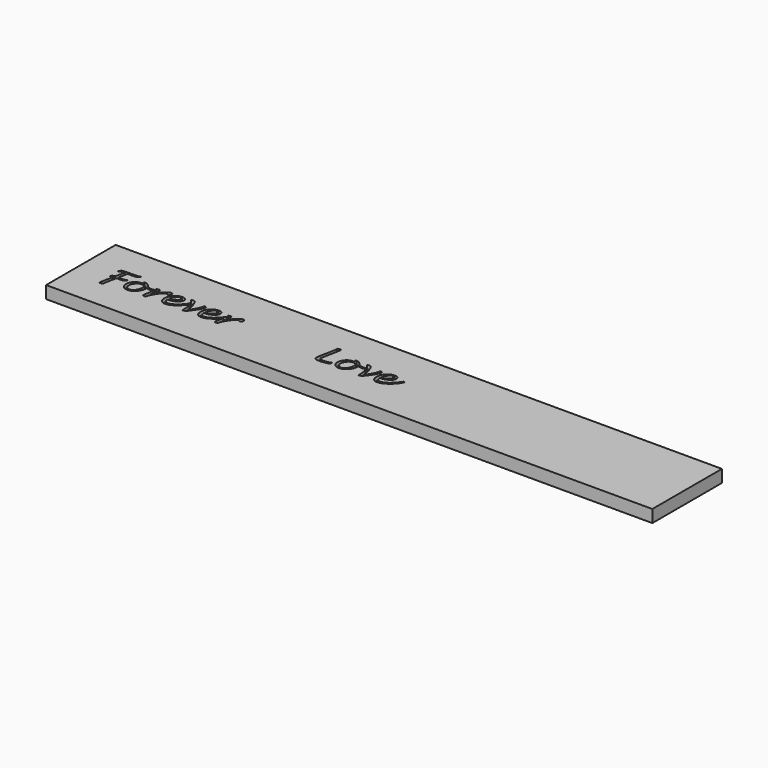
from build123d import *

# Parameters (mm, degrees)
F0_W     = 774.7
F0_H     = 111.125
F1_DEPTH = 15.875
F3_DEPTH = 4.7625


# Not quite as in the source:
# - ends of sketch curves that miss each other by under 0.0002 mm in the source are joined


with BuildPart() as f1:
    # F0 (on Top) → F1 (new body)
    with BuildSketch(Plane.XY):
        with Locations((387.35, 55.5625)):
            Rectangle(F0_W, F0_H)
    extrude(amount=F1_DEPTH)

    # F2 (on face) → F3 (cut)
    with BuildSketch(Plane.XY.offset(15.875)):
        with BuildLine():
            add(Edge.make_bspline(
                [(42.8841666709, 41.7124110682), (42.6348402709, 40.4654742682), (42.5101770709, 39.6582368682), (42.5101770709, 39.2906988682)],
                knots=[0, 0, 0, 0, 1, 1, 1, 1], degree=3))
            Line((42.8841666709, 41.7124110682), (45.6012046709, 55.3173368682))
            Line((45.6012046709, 55.3173368682), (49.8541806709, 55.3177940682))
            add(Edge.make_bspline(
                [(54.6779454709, 55.9281052682), (53.8641548709, 55.5212226682), (52.2562078709, 55.3177940682), (49.8541806709, 55.3177940682)],
                knots=[0, 0, 0, 0, 1, 1, 1, 1], degree=3))
            add(Edge.make_bspline(
                [(56.8633868709, 58.7633040682), (56.2333398709, 57.2800964682), (55.5048678709, 56.3350386682), (54.6779454709, 55.9281052682)],
                knots=[0, 0, 0, 0, 1, 1, 1, 1], degree=3))
            add(Edge.make_bspline(
                [(50.3266968709, 57.7591658682), (52.9649948709, 57.7591658682), (55.1438830709, 58.0938616682), (56.8633868709, 58.7633040682)],
                knots=[0, 0, 0, 0, 1, 1, 1, 1], degree=3))
            Line((50.3266968709, 57.7591658682), (46.0739240709, 57.7591658682))
            Line((46.0739240709, 57.7591658682), (48.4169216709, 69.5330310682))
            Line((48.4169216709, 69.5330310682), (54.4416492709, 69.5330310682))
            Line((54.4416492709, 69.5330310682), (56.1742594709, 69.5128634682))
            add(Edge.make_bspline(
                [(60.2498164709, 70.2216758682), (59.3704176709, 69.7491342682), (58.0118986709, 69.5128634682), (56.1742594709, 69.5128634682)],
                knots=[0, 0, 0, 0, 1, 1, 1, 1], degree=3))
            add(Edge.make_bspline(
                [(62.8093744709, 73.0962192682), (61.9955838709, 71.6655134682), (61.1423978709, 70.7073492682), (60.2498164709, 70.2216758682)],
                knots=[0, 0, 0, 0, 1, 1, 1, 1], degree=3))
            add(Edge.make_bspline(
                [(53.1815806709, 72.0724468682), (57.0405772709, 72.0724468682), (60.2498418709, 72.4136958682), (62.8093744709, 73.0962192682)],
                knots=[0, 0, 0, 0, 1, 1, 1, 1], degree=3))
            Line((53.1815806709, 72.0724468682), (48.0034604709, 72.0724468682))
            add(Edge.make_bspline(
                [(39.6948156709, 71.3439494682), (40.5873462709, 71.8296228682), (43.3569114709, 72.0724468682), (48.0034604709, 72.0724468682)],
                knots=[0, 0, 0, 0, 1, 1, 1, 1], degree=3))
            add(Edge.make_bspline(
                [(37.0368580709, 67.1896270682), (37.5487442709, 69.2634862682), (38.4347470709, 70.6482688682), (39.6948156709, 71.3439494682)],
                knots=[0, 0, 0, 0, 1, 1, 1, 1], degree=3))
            add(Edge.make_bspline(
                [(43.8687976709, 69.5325738682), (41.0073860709, 69.5325738682), (38.7300728709, 68.7516000682), (37.0368580709, 67.1896270682)],
                knots=[0, 0, 0, 0, 1, 1, 1, 1], degree=3))
            Line((43.8687976709, 69.5325738682), (44.3017660709, 69.5325738682))
            Line((44.3017660709, 69.5325738682), (41.9391088709, 57.7587086682))
            Line((41.9391088709, 57.7587086682), (41.4075122709, 57.7587086682))
            add(Edge.make_bspline(
                [(39.0448804709, 57.1483720682), (39.5436602709, 57.5552546682), (40.3312126709, 57.7587086682), (41.4075122709, 57.7587086682)],
                knots=[0, 0, 0, 0, 1, 1, 1, 1], degree=3))
            add(Edge.make_bspline(
                [(37.3516656709, 54.4707040682), (37.9948190709, 55.8620398682), (38.5592070709, 56.7545958682), (39.0448804709, 57.1483720682)],
                knots=[0, 0, 0, 0, 1, 1, 1, 1], degree=3))
            add(Edge.make_bspline(
                [(41.1712668709, 55.3173368682), (39.9899636709, 55.3173368682), (38.7167632709, 55.0351174682), (37.3516656709, 54.4707040682)],
                knots=[0, 0, 0, 0, 1, 1, 1, 1], degree=3))
            Line((41.1712668709, 55.3173368682), (41.4666434709, 55.3173368682))
            Line((41.4666434709, 55.3173368682), (38.4936496709, 40.3735516682))
            add(Edge.make_bspline(
                [(38.1000004709, 37.9321798682), (38.1000004709, 38.2208254682), (38.2312168709, 39.0346160682), (38.4936496709, 40.3735516682)],
                knots=[0, 0, 0, 0, 1, 1, 1, 1], degree=3))
            add(Edge.make_bspline(
                [(39.1238490709, 37.1052828682), (38.4413002709, 37.1052828682), (38.1000004709, 37.3808982682), (38.1000004709, 37.9321798682)],
                knots=[0, 0, 0, 0, 1, 1, 1, 1], degree=3))
            add(Edge.make_bspline(
                [(42.7662344709, 38.1093956682), (41.4405322709, 37.4399786682), (40.2264122709, 37.1052828682), (39.1238490709, 37.1052828682)],
                knots=[0, 0, 0, 0, 1, 1, 1, 1], degree=3))
            add(Edge.make_bspline(
                [(42.5101770709, 39.2906988682), (42.5101770709, 38.9231862682), (42.5955210709, 38.5294354682), (42.7662344709, 38.1093956682)],
                knots=[0, 0, 0, 0, 1, 1, 1, 1], degree=3))
        make_face()
        with BuildLine():
            add(Edge.make_bspline(
                [(82.6554564739, 57.4433294306), (82.6947450052, 57.1286193013), (82.7143892709, 56.8465227238), (82.7143892709, 56.5970650682)],
                knots=[0.0003900722, 0.0003900722, 0.0003900722, 0.0003900722, 1, 1, 1, 1], degree=3))
            add(Edge.make_bspline(
                [(87.6166400709, 56.5377814682), (86.1597881245, 56.5377814682), (84.5060602589, 56.8396477192), (82.6554564739, 57.4433294306)],
                knots=[0, 0, 0, 0, 0.9999368173, 0.9999368173, 0.9999368173, 0.9999368173], degree=3))
            add(Edge.make_bspline(
                [(91.5525691041, 57.3439651685), (90.2599710329, 56.8065131621), (88.9479984823, 56.5377814682), (87.6166400709, 56.5377814682)],
                knots=[0.3926410414, 0.3926410414, 0.3926410414, 0.3926410414, 1, 1, 1, 1], degree=3))
            add(Edge.make_bspline(
                [(91.5525691041, 57.3439651685), (91.6859533121, 58.2821458932), (91.7633692368, 59.0804045786), (91.7848148506, 59.7387412247)],
                knots=[0.4869393533, 0.4869393533, 0.4869393533, 0.4869393533, 0.9175112155, 0.9175112155, 0.9175112155, 0.9175112155], degree=3))
            add(Edge.make_bspline(
                [(88.0695220709, 58.8413582682), (89.2360031141, 58.8413582682), (90.4744377518, 59.1404859201), (91.7848148529, 59.7387412239)],
                knots=[0, 0, 0, 0, 0.7595714679, 0.7595714679, 0.7595714679, 0.7595714679], degree=3))
            add(Edge.make_bspline(
                [(81.2571912709, 61.0661696682), (83.4360794709, 59.5829620682), (85.7068648709, 58.8413582682), (88.0695220709, 58.8413582682)],
                knots=[0, 0, 0, 0, 1, 1, 1, 1], degree=3))
            add(Edge.make_bspline(
                [(73.2636080709, 65.9883848682), (76.4662686709, 65.7259520682), (79.1308048709, 64.0852136682), (81.2571912709, 61.0661696682)],
                knots=[0, 0, 0, 0, 1, 1, 1, 1], degree=3))
            add(Edge.make_bspline(
                [(72.6138506709, 64.1769838682), (72.6138506709, 64.8070308682), (72.8304364709, 65.4108142682), (73.2636080709, 65.9883848682)],
                knots=[0, 0, 0, 0, 1, 1, 1, 1], degree=3))
            add(Edge.make_bspline(
                [(73.1062804709, 62.6806698682), (72.7780108709, 63.2713214682), (72.6138506709, 63.7701012682), (72.6138506709, 64.1769838682)],
                knots=[0, 0, 0, 0, 1, 1, 1, 1], degree=3))
            add(Edge.make_bspline(
                [(71.6887064709, 62.8580888682), (72.1349844709, 62.8580888682), (72.6075006709, 62.7989576682), (73.1062804709, 62.6806698682)],
                knots=[0, 0, 0, 0, 1, 1, 1, 1], degree=3))
            add(Edge.make_bspline(
                [(64.0888232709, 59.4913188682), (66.2414732709, 61.7358406682), (68.7747676709, 62.8580888682), (71.6887064709, 62.8580888682)],
                knots=[0, 0, 0, 0, 1, 1, 1, 1], degree=3))
            add(Edge.make_bspline(
                [(60.8795586709, 51.5371056682), (60.8795586709, 54.5953926682), (61.9493050709, 57.2467970682), (64.0888232709, 59.4913188682)],
                knots=[0, 0, 0, 0, 1, 1, 1, 1], degree=3))
            add(Edge.make_bspline(
                [(63.3603512709, 44.9610456682), (61.7064810709, 46.6542858682), (60.8795586709, 48.8463058682), (60.8795586709, 51.5371056682)],
                knots=[0, 0, 0, 0, 1, 1, 1, 1], degree=3))
            add(Edge.make_bspline(
                [(69.8182504709, 42.4408830682), (67.1799778709, 42.4408830682), (65.0273532709, 43.2809372682), (63.3603512709, 44.9610456682)],
                knots=[0, 0, 0, 0, 1, 1, 1, 1], degree=3))
            add(Edge.make_bspline(
                [(78.8553672709, 46.6739454682), (76.2827282709, 43.8519038682), (73.2703644709, 42.4408830682), (69.8182504709, 42.4408830682)],
                knots=[0, 0, 0, 0, 1, 1, 1, 1], degree=3))
            add(Edge.make_bspline(
                [(82.7143892709, 56.5970650682), (82.7143892709, 52.8037274682), (81.4280570709, 49.4960124682), (78.8553672709, 46.6739454682)],
                knots=[0, 0, 0, 0, 1, 1, 1, 1], degree=3))
        make_face()
        with BuildLine():
            add(Edge.make_bspline(
                [(78.1860772709, 59.1172276682), (77.0966204709, 59.4455226682), (76.0924822709, 59.9705406682), (75.1736880709, 60.6923324682)],
                knots=[0, 0, 0, 0, 1, 1, 1, 1], degree=3))
            add(Edge.make_bspline(
                [(78.6979634709, 55.9868808682), (78.6979634709, 57.0631573052), (78.5273416686, 58.1065945057), (78.1860772709, 59.1172276682)],
                knots=[0, 0, 0, 0, 0.9999548807, 0.9999548807, 0.9999548807, 0.9999548807], degree=3))
            add(Edge.make_bspline(
                [(76.2959616709, 47.9735872682), (77.8973046709, 50.2181090682), (78.6979634709, 52.8891984682), (78.6979634709, 55.9868808682)],
                knots=[0, 0, 0, 0, 1, 1, 1, 1], degree=3))
            add(Edge.make_bspline(
                [(70.5665344709, 44.6264768682), (72.7847926709, 44.6264768682), (74.6946186709, 45.7421718682), (76.2959616709, 47.9735872682)],
                knots=[0, 0, 0, 0, 1, 1, 1, 1], degree=3))
            add(Edge.make_bspline(
                [(66.5303474709, 46.4181674682), (67.5804088709, 45.2237070682), (68.9257960709, 44.6264768682), (70.5665344709, 44.6264768682)],
                knots=[0, 0, 0, 0, 1, 1, 1, 1], degree=3))
            add(Edge.make_bspline(
                [(64.9749022709, 51.0253464682), (64.9749022709, 49.1614690682), (65.4933924709, 47.6257596682), (66.5303474709, 46.4181674682)],
                knots=[0, 0, 0, 0, 1, 1, 1, 1], degree=3))
            add(Edge.make_bspline(
                [(67.5541452709, 57.8967068682), (65.8346414709, 55.8884558682), (64.9749022709, 53.5979854682), (64.9749022709, 51.0253464682)],
                knots=[0, 0, 0, 0, 1, 1, 1, 1], degree=3))
            add(Edge.make_bspline(
                [(73.5001328709, 60.9090452682), (71.2687682709, 60.9090452682), (69.2867554709, 59.9049324682), (67.5541452709, 57.8967068682)],
                knots=[0, 0, 0, 0, 1, 1, 1, 1], degree=3))
            add(Edge.make_bspline(
                [(75.1736880709, 60.6923324682), (74.5042456709, 60.8368076682), (73.9464108709, 60.9090452682), (73.5001328709, 60.9090452682)],
                knots=[0, 0, 0, 0, 1, 1, 1, 1], degree=3))
        make_face(mode=Mode.SUBTRACT)
        with BuildLine():
            add(Edge.make_bspline(
                [(91.5525691041, 57.3439651685), (91.6859533121, 58.2821458932), (91.7633692368, 59.0804045786), (91.7848148506, 59.7387412247)],
                knots=[0.4869393533, 0.4869393533, 0.4869393533, 0.4869393533, 0.9175112155, 0.9175112155, 0.9175112155, 0.9175112155], degree=3))
            add(Edge.make_bspline(
                [(94.0351692709, 58.7232228682), (93.2157309513, 58.1511668589), (92.3881985874, 57.6914132673), (91.5525691041, 57.3439651685)],
                knots=[0, 0, 0, 0, 0.3926410414, 0.3926410414, 0.3926410414, 0.3926410414], degree=3))
            Line((94.0351692709, 58.7232228682), (93.0507668709, 60.3967526682))
            add(Edge.make_bspline(
                [(91.7848148529, 59.7387412239), (92.1995908894, 59.9281080585), (92.6215750131, 60.1474452066), (93.0507668709, 60.3967526682)],
                knots=[0.7595714679, 0.7595714679, 0.7595714679, 0.7595714679, 1, 1, 1, 1], degree=3))
        make_face()
        with BuildLine():
            add(Edge.make_bspline(
                [(94.0351692709, 58.7232228682), (93.2157309513, 58.1511668589), (92.3881985874, 57.6914132673), (91.5525691041, 57.3439651685)],
                knots=[0, 0, 0, 0, 0.3926410414, 0.3926410414, 0.3926410414, 0.3926410414], degree=3))
            add(Edge.make_bspline(
                [(90.8852898709, 53.6240966682), (91.1792957692, 55.0430081431), (91.4017231579, 56.2829643099), (91.5525691041, 57.3439651685)],
                knots=[0, 0, 0, 0, 0.4869393533, 0.4869393533, 0.4869393533, 0.4869393533], degree=3))
            Line((90.8852898709, 53.6240966682), (89.9008620709, 48.7215664682))
            add(Edge.make_bspline(
                [(89.1920496709, 44.2128632682), (89.1920496709, 44.8166720682), (89.4283204709, 46.3195646682), (89.9008620709, 48.7215664682)],
                knots=[0, 0, 0, 0, 1, 1, 1, 1], degree=3))
            add(Edge.make_bspline(
                [(91.2003006709, 42.4408830682), (89.8614666709, 42.4408830682), (89.1920496709, 43.0315600682), (89.1920496709, 44.2128632682)],
                knots=[0, 0, 0, 0, 1, 1, 1, 1], degree=3))
            add(Edge.make_bspline(
                [(93.3463720709, 43.0709300682), (92.4538414709, 42.6509156682), (91.7384758709, 42.4408830682), (91.2003006709, 42.4408830682)],
                knots=[0, 0, 0, 0, 1, 1, 1, 1], degree=3))
            Line((93.3463720709, 43.0709300682), (93.3266616709, 43.4056512682))
            add(Edge.make_bspline(
                [(95.0986926709, 48.4065556682), (93.9173386709, 46.0701620682), (93.3266616709, 44.4032108682), (93.3266616709, 43.4056512682)],
                knots=[0, 0, 0, 0, 1, 1, 1, 1], degree=3))
            add(Edge.make_bspline(
                [(99.2726746709, 55.2385460682), (97.6713316709, 53.0334196682), (96.2799958709, 50.7560810682), (95.0986926709, 48.4065556682)],
                knots=[0, 0, 0, 0, 1, 1, 1, 1], degree=3))
            add(Edge.make_bspline(
                [(105.6518338709, 60.5545120682), (103.9848318709, 60.5545120682), (101.8584454709, 58.7825318682), (99.2726746709, 55.2385460682)],
                knots=[0, 0, 0, 0, 1, 1, 1, 1], degree=3))
            add(Edge.make_bspline(
                [(107.7781948709, 58.9991176682), (107.2794150709, 60.0360472682), (106.5706280709, 60.5545120682), (105.6518338709, 60.5545120682)],
                knots=[0, 0, 0, 0, 1, 1, 1, 1], degree=3))
            add(Edge.make_bspline(
                [(110.7708736709, 62.6612134682), (110.7708736709, 61.7423938682), (109.7733140709, 60.5216952682), (107.7781948709, 58.9991176682)],
                knots=[0, 0, 0, 0, 1, 1, 1, 1], degree=3))
            add(Edge.make_bspline(
                [(109.9833466709, 64.1575274682), (110.5083646709, 63.7506448682), (110.7708736709, 63.2518650682), (110.7708736709, 62.6612134682)],
                knots=[0, 0, 0, 0, 1, 1, 1, 1], degree=3))
            add(Edge.make_bspline(
                [(108.1129160709, 64.7875744682), (108.8348348709, 64.7875744682), (109.4583032709, 64.5775672682), (109.9833466709, 64.1575274682)],
                knots=[0, 0, 0, 0, 1, 1, 1, 1], degree=3))
            add(Edge.make_bspline(
                [(101.2612152709, 60.7710978682), (103.7813778709, 63.4487404682), (106.0652696709, 64.7875744682), (108.1129160709, 64.7875744682)],
                knots=[0, 0, 0, 0, 1, 1, 1, 1], degree=3))
            add(Edge.make_bspline(
                [(93.7795436709, 49.5485396682), (96.2603108709, 54.3657004682), (98.7542098709, 58.1065616682), (101.2612152709, 60.7710978682)],
                knots=[0, 0, 0, 0, 1, 1, 1, 1], degree=3))
            Line((93.7795436709, 49.5485396682), (94.9017664709, 55.2779668682))
            add(Edge.make_bspline(
                [(95.8862450709, 60.9679732682), (95.8862450709, 60.2460798682), (95.5580770709, 58.3493856682), (94.9017664709, 55.2779668682)],
                knots=[0, 0, 0, 0, 1, 1, 1, 1], degree=3))
            add(Edge.make_bspline(
                [(94.5080156709, 62.7202938682), (95.4268352709, 62.7202938682), (95.8862450709, 62.1361954682), (95.8862450709, 60.9679732682)],
                knots=[0, 0, 0, 0, 1, 1, 1, 1], degree=3))
            add(Edge.make_bspline(
                [(91.1412456709, 62.0114814682), (92.5194496709, 62.4840230682), (93.6417232709, 62.7202938682), (94.5080156709, 62.7202938682)],
                knots=[0, 0, 0, 0, 1, 1, 1, 1], degree=3))
            add(Edge.make_bspline(
                [(91.7909776709, 60.1017062682), (91.7909776709, 60.8629950682), (91.5743918709, 61.4995698682), (91.1412456709, 62.0114814682)],
                knots=[0, 0, 0, 0, 1, 1, 1, 1], degree=3))
            add(Edge.make_bspline(
                [(91.7848148506, 59.7387412247), (91.7889233927, 59.8648650952), (91.7909776709, 59.985853443), (91.7909776709, 60.1017062682)],
                knots=[0.9175112155, 0.9175112155, 0.9175112155, 0.9175112155, 1, 1, 1, 1], degree=3))
            add(Edge.make_bspline(
                [(91.7848148529, 59.7387412239), (92.1995908894, 59.9281080585), (92.6215750131, 60.1474452066), (93.0507668709, 60.3967526682)],
                knots=[0.7595714679, 0.7595714679, 0.7595714679, 0.7595714679, 1, 1, 1, 1], degree=3))
            Line((93.0507668709, 60.3967526682), (94.0351692709, 58.7232228682))
        make_face()
        with BuildLine():
            add(Edge.make_bspline(
                [(114.3542548709, 51.1236444682), (114.3542548709, 47.2777796682), (115.9818360709, 45.3548472682), (119.2370492709, 45.3548472682)],
                knots=[0, 0, 0, 0, 1, 1, 1, 1], degree=3))
            add(Edge.make_bspline(
                [(124.1001332709, 53.8406824682), (121.2780916709, 52.0293068682), (118.0294824709, 51.1236444682), (114.3542548709, 51.1236444682)],
                knots=[0, 0, 0, 0, 1, 1, 1, 1], degree=3))
            add(Edge.make_bspline(
                [(128.3529060709, 60.0819958682), (128.3529060709, 57.7324704682), (126.9353066709, 55.6520326682), (124.1001332709, 53.8406824682)],
                knots=[0, 0, 0, 0, 1, 1, 1, 1], degree=3))
            add(Edge.make_bspline(
                [(126.8172220709, 63.5078462682), (127.8410198709, 62.6546602682), (128.3529060709, 61.5127016682), (128.3529060709, 60.0819958682)],
                knots=[0, 0, 0, 0, 1, 1, 1, 1], degree=3))
            add(Edge.make_bspline(
                [(122.7613246709, 64.7875744682), (124.4545394709, 64.7875744682), (125.8065052709, 64.3610068682), (126.8172220709, 63.5078462682)],
                knots=[0, 0, 0, 0, 1, 1, 1, 1], degree=3))
            add(Edge.make_bspline(
                [(113.7635778709, 60.7317278682), (116.2574768709, 63.4356340682), (119.2567342709, 64.7875744682), (122.7613246709, 64.7875744682)],
                knots=[0, 0, 0, 0, 1, 1, 1, 1], degree=3))
            add(Edge.make_bspline(
                [(110.0424016709, 50.9661390682), (110.0424016709, 54.7726084682), (111.2827852709, 58.0278216682), (113.7635778709, 60.7317278682)],
                knots=[0, 0, 0, 0, 1, 1, 1, 1], degree=3))
            add(Edge.make_bspline(
                [(112.0900226709, 44.7248002682), (110.7249504709, 46.2473778682), (110.0424016709, 48.3278410682), (110.0424016709, 50.9661390682)],
                knots=[0, 0, 0, 0, 1, 1, 1, 1], degree=3))
            add(Edge.make_bspline(
                [(117.7013144709, 42.4408830682), (115.3386826709, 42.4408830682), (113.4682520709, 43.2021972682), (112.0900226709, 44.7248002682)],
                knots=[0, 0, 0, 0, 1, 1, 1, 1], degree=3))
            add(Edge.make_bspline(
                [(129.3963888709, 47.1661974682), (125.2880404709, 44.0159878682), (121.3896738709, 42.4408830682), (117.7013144709, 42.4408830682)],
                knots=[0, 0, 0, 0, 1, 1, 1, 1], degree=3))
            add(Edge.make_bspline(
                [(137.9029661131, 56.4732409138), (135.5778224369, 52.8259102249), (132.7423012193, 49.7235578799), (129.3963888709, 47.1661974682)],
                knots=[0.1881870236, 0.1881870236, 0.1881870236, 0.1881870236, 1, 1, 1, 1], degree=3))
            add(Edge.make_bspline(
                [(137.9029661131, 56.4732409138), (137.6078076226, 57.2942126627), (137.3020171195, 58.071776328), (136.9855946038, 58.8059316671)],
                knots=[0.0281384142, 0.0281384142, 0.0281384142, 0.0281384142, 0.2402573175, 0.2402573175, 0.2402573175, 0.2402573175], degree=3))
            add(Edge.make_bspline(
                [(128.5694918709, 49.3910342682), (131.6496232223, 51.8289595446), (134.4549845028, 54.9672586776), (136.9855946038, 58.8059316671)],
                knots=[0, 0, 0, 0, 0.9060310951, 0.9060310951, 0.9060310951, 0.9060310951], degree=3))
            add(Edge.make_bspline(
                [(119.2370492709, 45.3548472682), (122.0590908709, 45.3548472682), (125.1699050709, 46.7002344682), (128.5694918709, 49.3910342682)],
                knots=[0, 0, 0, 0, 1, 1, 1, 1], degree=3))
        make_face()
        with BuildLine():
            add(Edge.make_bspline(
                [(114.5115062709, 53.0137600682), (117.2548078709, 53.1582352682), (119.6043332709, 53.9457876682), (121.5600824709, 55.3763918682)],
                knots=[0, 0, 0, 0, 1, 1, 1, 1], degree=3))
            add(Edge.make_bspline(
                [(117.3269692709, 59.9835454682), (115.8174980709, 58.0671916682), (114.8790188709, 55.7439298682), (114.5115062709, 53.0137600682)],
                knots=[0, 0, 0, 0, 1, 1, 1, 1], degree=3))
            add(Edge.make_bspline(
                [(122.2688440709, 62.8580888682), (120.4837320709, 62.8580888682), (118.8364404709, 61.8998992682), (117.3269692709, 59.9835454682)],
                knots=[0, 0, 0, 0, 1, 1, 1, 1], degree=3))
            add(Edge.make_bspline(
                [(124.5133404709, 60.3379262682), (124.5133404709, 62.0180346682), (123.7651834709, 62.8580888682), (122.2688440709, 62.8580888682)],
                knots=[0, 0, 0, 0, 1, 1, 1, 1], degree=3))
            add(Edge.make_bspline(
                [(121.5600824709, 55.3763918682), (123.5289126709, 56.8071230682), (124.5133404709, 58.4609678682), (124.5133404709, 60.3379262682)],
                knots=[0, 0, 0, 0, 1, 1, 1, 1], degree=3))
        make_face(mode=Mode.SUBTRACT)
        with BuildLine():
            add(Edge.make_bspline(
                [(136.9855946038, 58.8059316671), (135.8522694395, 61.4354434087), (134.5825519952, 63.5080934552), (133.1764422709, 65.0238706682)],
                knots=[0.2402573175, 0.2402573175, 0.2402573175, 0.2402573175, 1, 1, 1, 1], degree=3))
            add(Edge.make_bspline(
                [(136.9855946038, 58.8059316671), (137.2480565227, 59.2040591695), (137.5075630047, 59.6097204365), (137.7641140709, 60.0229154682)],
                knots=[0.9060310951, 0.9060310951, 0.9060310951, 0.9060310951, 1, 1, 1, 1], degree=3))
            Line((137.7641140709, 60.0229154682), (139.4376692709, 59.0975680682))
            add(Edge.make_bspline(
                [(139.4376692709, 59.0975680682), (138.9535272147, 58.1935073695), (138.4419595519, 57.3187315949), (137.9029661131, 56.4732409138)],
                knots=[0, 0, 0, 0, 0.1881870236, 0.1881870236, 0.1881870236, 0.1881870236], degree=3))
            add(Edge.make_bspline(
                [(138.0198666709, 56.1442338682), (137.9810869106, 56.2546667383), (137.942120058, 56.3643357537), (137.9029661131, 56.4732409138)],
                knots=[0, 0, 0, 0, 0.0281384142, 0.0281384142, 0.0281384142, 0.0281384142], degree=3))
            add(Edge.make_bspline(
                [(140.0871980709, 45.3942172682), (140.0871980709, 48.6362732682), (139.3980960709, 52.2196290682), (138.0198666709, 56.1442338682)],
                knots=[0, 0, 0, 0, 1, 1, 1, 1], degree=3))
            add(Edge.make_bspline(
                [(139.6542296709, 42.4015384682), (139.9428752709, 43.5566034682), (140.0871980709, 44.5541630682), (140.0871980709, 45.3942172682)],
                knots=[0, 0, 0, 0, 1, 1, 1, 1], degree=3))
            add(Edge.make_bspline(
                [(143.3161222709, 43.1890908682), (142.5810970515, 42.7953028658), (141.3604827679, 42.5327983968), (139.6542296709, 42.4015384682)],
                knots=[0, 0, 0, 0, 0.9999654709, 0.9999654709, 0.9999654709, 0.9999654709], degree=3))
            add(Edge.make_bspline(
                [(146.0332110709, 45.8273888682), (144.9568606709, 44.4622912682), (144.0511728709, 43.5828670682), (143.3161222709, 43.1890908682)],
                knots=[0, 0, 0, 0, 1, 1, 1, 1], degree=3))
            add(Edge.make_bspline(
                [(152.1563890709, 54.7660298682), (150.2794052709, 51.6158202682), (148.2383374709, 48.6362732682), (146.0332110709, 45.8273888682)],
                knots=[0, 0, 0, 0, 1, 1, 1, 1], degree=3))
            add(Edge.make_bspline(
                [(154.9915624709, 60.8301782682), (154.9915624709, 59.9375968682), (154.0465046709, 57.9162140682), (152.1563890709, 54.7660298682)],
                knots=[0, 0, 0, 0, 1, 1, 1, 1], degree=3))
            add(Edge.make_bspline(
                [(152.0382282709, 63.5078462682), (154.0071092709, 62.7202684682), (154.9915624709, 61.8277124682), (154.9915624709, 60.8301782682)],
                knots=[0, 0, 0, 0, 1, 1, 1, 1], degree=3))
            add(Edge.make_bspline(
                [(149.4984314709, 55.4945018682), (150.9947708709, 58.5922096682), (151.8413528709, 61.2633244682), (152.0382282709, 63.5078462682)],
                knots=[0, 0, 0, 0, 1, 1, 1, 1], degree=3))
            add(Edge.make_bspline(
                [(143.8083742709, 46.4770700682), (146.1053724709, 49.3910088682), (148.0020666709, 52.3968194682), (149.4984314709, 55.4945018682)],
                knots=[0, 0, 0, 0, 1, 1, 1, 1], degree=3))
            add(Edge.make_bspline(
                [(140.6187946709, 60.2001312682), (142.1020022709, 56.4199000682), (143.1651954709, 51.8455378682), (143.8083742709, 46.4770700682)],
                knots=[0, 0, 0, 0, 1, 1, 1, 1], degree=3))
            add(Edge.make_bspline(
                [(136.2478864709, 65.8901376682), (137.6917494709, 65.8901376682), (139.1487188709, 63.9934688682), (140.6187946709, 60.2001312682)],
                knots=[0, 0, 0, 0, 1, 1, 1, 1], degree=3))
            add(Edge.make_bspline(
                [(133.1764422709, 65.0238706682), (134.3184008709, 65.6013904682), (135.3422240709, 65.8901376682), (136.2478864709, 65.8901376682)],
                knots=[0, 0, 0, 0, 1, 1, 1, 1], degree=3))
        make_face()
        with BuildLine():
            add(Edge.make_bspline(
                [(136.9855946038, 58.8059316671), (137.2480565227, 59.2040591695), (137.5075630047, 59.6097204365), (137.7641140709, 60.0229154682)],
                knots=[0.9060310951, 0.9060310951, 0.9060310951, 0.9060310951, 1, 1, 1, 1], degree=3))
            add(Edge.make_bspline(
                [(137.9029661131, 56.4732409138), (137.6078076226, 57.2942126627), (137.3020171195, 58.071776328), (136.9855946038, 58.8059316671)],
                knots=[0.0281384142, 0.0281384142, 0.0281384142, 0.0281384142, 0.2402573175, 0.2402573175, 0.2402573175, 0.2402573175], degree=3))
            add(Edge.make_bspline(
                [(139.4376692709, 59.0975680682), (138.9535272147, 58.1935073695), (138.4419595519, 57.3187315949), (137.9029661131, 56.4732409138)],
                knots=[0, 0, 0, 0, 0.1881870236, 0.1881870236, 0.1881870236, 0.1881870236], degree=3))
            Line((139.4376692709, 59.0975680682), (137.7641140709, 60.0229154682))
        make_face()
        with BuildLine():
            add(Edge.make_bspline(
                [(160.7408524709, 51.1236444682), (160.7408524709, 47.2777796682), (162.3684336709, 45.3548472682), (165.6236468709, 45.3548472682)],
                knots=[0, 0, 0, 0, 1, 1, 1, 1], degree=3))
            add(Edge.make_bspline(
                [(170.4867816709, 53.8406824682), (167.6647146709, 52.0293068682), (164.4160800709, 51.1236444682), (160.7408524709, 51.1236444682)],
                knots=[0, 0, 0, 0, 1, 1, 1, 1], degree=3))
            add(Edge.make_bspline(
                [(174.7395544709, 60.0819958682), (174.7395544709, 57.7324704682), (173.3219550709, 55.6520326682), (170.4867816709, 53.8406824682)],
                knots=[0, 0, 0, 0, 1, 1, 1, 1], degree=3))
            add(Edge.make_bspline(
                [(173.2038196709, 63.5078462682), (174.2276428709, 62.6546602682), (174.7395544709, 61.5127016682), (174.7395544709, 60.0819958682)],
                knots=[0, 0, 0, 0, 1, 1, 1, 1], degree=3))
            add(Edge.make_bspline(
                [(169.1479222709, 64.7875744682), (170.8411878709, 64.7875744682), (172.1931282709, 64.3610068682), (173.2038196709, 63.5078462682)],
                knots=[0, 0, 0, 0, 1, 1, 1, 1], degree=3))
            add(Edge.make_bspline(
                [(160.1502262709, 60.7317278682), (162.6440998709, 63.4356340682), (165.6433318709, 64.7875744682), (169.1479222709, 64.7875744682)],
                knots=[0, 0, 0, 0, 1, 1, 1, 1], degree=3))
            add(Edge.make_bspline(
                [(156.4290500709, 50.9661390682), (156.4290500709, 54.7726084682), (157.6694336709, 58.0278216682), (160.1502262709, 60.7317278682)],
                knots=[0, 0, 0, 0, 1, 1, 1, 1], degree=3))
            add(Edge.make_bspline(
                [(158.4766964709, 44.7248002682), (157.1115988709, 46.2473778682), (156.4290500709, 48.3278410682), (156.4290500709, 50.9661390682)],
                knots=[0, 0, 0, 0, 1, 1, 1, 1], degree=3))
            add(Edge.make_bspline(
                [(164.0879628709, 42.4408830682), (161.7253056709, 42.4408830682), (159.8548750709, 43.2021972682), (158.4766964709, 44.7248002682)],
                knots=[0, 0, 0, 0, 1, 1, 1, 1], degree=3))
            add(Edge.make_bspline(
                [(175.7830626709, 47.1661974682), (171.6746634709, 44.0159878682), (167.7762968709, 42.4408830682), (164.0879628709, 42.4408830682)],
                knots=[0, 0, 0, 0, 1, 1, 1, 1], degree=3))
            add(Edge.make_bspline(
                [(182.8709229566, 54.4013877377), (180.8390008071, 51.6365223504), (178.4763807119, 49.2247898978), (175.7830626709, 47.1661974682)],
                knots=[0.346516807, 0.346516807, 0.346516807, 0.346516807, 1, 1, 1, 1], degree=3))
            add(Edge.make_bspline(
                [(182.8709229566, 54.4013877377), (183.2551515805, 56.3452029353), (183.4913943444, 57.9190913878), (183.5796686801, 59.1230530952)],
                knots=[0.0910643098, 0.0910643098, 0.0910643098, 0.0910643098, 0.7911649064, 0.7911649064, 0.7911649064, 0.7911649064], degree=3))
            add(Edge.make_bspline(
                [(174.9561402709, 49.3910342682), (178.120668564, 51.8957597599), (180.9951848628, 55.1397660356), (183.5796686801, 59.1230530952)],
                knots=[0, 0, 0, 0, 0.9308567421, 0.9308567421, 0.9308567421, 0.9308567421], degree=3))
            add(Edge.make_bspline(
                [(165.6236468709, 45.3548472682), (168.4457138709, 45.3548472682), (171.5565534709, 46.7002344682), (174.9561402709, 49.3910342682)],
                knots=[0, 0, 0, 0, 1, 1, 1, 1], degree=3))
        make_face()
        with BuildLine():
            add(Edge.make_bspline(
                [(160.8981038709, 53.0137600682), (163.6414054709, 53.1582352682), (165.9909308709, 53.9457876682), (167.9466800709, 55.3763918682)],
                knots=[0, 0, 0, 0, 1, 1, 1, 1], degree=3))
            add(Edge.make_bspline(
                [(163.7136176709, 59.9835454682), (162.2041464709, 58.0671916682), (161.2656418709, 55.7439298682), (160.8981038709, 53.0137600682)],
                knots=[0, 0, 0, 0, 1, 1, 1, 1], degree=3))
            add(Edge.make_bspline(
                [(168.6554924709, 62.8580888682), (166.8703804709, 62.8580888682), (165.2230888709, 61.8998992682), (163.7136176709, 59.9835454682)],
                knots=[0, 0, 0, 0, 1, 1, 1, 1], degree=3))
            add(Edge.make_bspline(
                [(170.8999888709, 60.3379262682), (170.8999888709, 62.0180346682), (170.1518318709, 62.8580888682), (168.6554924709, 62.8580888682)],
                knots=[0, 0, 0, 0, 1, 1, 1, 1], degree=3))
            add(Edge.make_bspline(
                [(167.9466800709, 55.3763918682), (169.9155610709, 56.8071230682), (170.8999888709, 58.4609678682), (170.8999888709, 60.3379262682)],
                knots=[0, 0, 0, 0, 1, 1, 1, 1], degree=3))
        make_face(mode=Mode.SUBTRACT)
        with BuildLine():
            add(Edge.make_bspline(
                [(183.5796686801, 59.1230530952), (183.6060002949, 59.4821864212), (183.6191658709, 59.8084041456), (183.6191658709, 60.1017062682)],
                knots=[0.7911649064, 0.7911649064, 0.7911649064, 0.7911649064, 1, 1, 1, 1], degree=3))
            add(Edge.make_bspline(
                [(183.5796686801, 59.1230530952), (183.7716419699, 59.4189283164), (183.9620150363, 59.7188824407), (184.1507878709, 60.0229154682)],
                knots=[0.9308567421, 0.9308567421, 0.9308567421, 0.9308567421, 1, 1, 1, 1], degree=3))
            Line((184.1507878709, 60.0229154682), (185.8243176709, 59.0975680682))
            add(Edge.make_bspline(
                [(185.8243176709, 59.0975680682), (184.932837416, 57.4328824769), (183.9483725112, 55.8674886811), (182.8709229566, 54.4013877377)],
                knots=[0, 0, 0, 0, 0.346516807, 0.346516807, 0.346516807, 0.346516807], degree=3))
            add(Edge.make_bspline(
                [(182.7134780709, 53.6240966682), (182.7684635025, 53.8894524937), (182.8209451182, 54.1485495169), (182.8709229566, 54.4013877377)],
                knots=[0, 0, 0, 0, 0.0910643098, 0.0910643098, 0.0910643098, 0.0910643098], degree=3))
            Line((182.7134780709, 53.6240966682), (181.7290502709, 48.7215664682))
            add(Edge.make_bspline(
                [(181.0202378709, 44.2128632682), (181.0202378709, 44.8166720682), (181.2565086709, 46.3195646682), (181.7290502709, 48.7215664682)],
                knots=[0, 0, 0, 0, 1, 1, 1, 1], degree=3))
            add(Edge.make_bspline(
                [(183.0284888709, 42.4408830682), (181.6896548709, 42.4408830682), (181.0202378709, 43.0315600682), (181.0202378709, 44.2128632682)],
                knots=[0, 0, 0, 0, 1, 1, 1, 1], degree=3))
            add(Edge.make_bspline(
                [(185.1745602709, 43.0709300682), (184.2820296709, 42.6509156682), (183.5666640709, 42.4408830682), (183.0284888709, 42.4408830682)],
                knots=[0, 0, 0, 0, 1, 1, 1, 1], degree=3))
            Line((185.1745602709, 43.0709300682), (185.1548498709, 43.4056512682))
            add(Edge.make_bspline(
                [(186.9268808709, 48.4065556682), (185.7455268709, 46.0701620682), (185.1548498709, 44.4032108682), (185.1548498709, 43.4056512682)],
                knots=[0, 0, 0, 0, 1, 1, 1, 1], degree=3))
            add(Edge.make_bspline(
                [(191.1008628709, 55.2385460682), (189.4995198709, 53.0334196682), (188.1081840709, 50.7560810682), (186.9268808709, 48.4065556682)],
                knots=[0, 0, 0, 0, 1, 1, 1, 1], degree=3))
            add(Edge.make_bspline(
                [(197.4800220709, 60.5545120682), (195.8130454709, 60.5545120682), (193.6866336709, 58.7825318682), (191.1008628709, 55.2385460682)],
                knots=[0, 0, 0, 0, 1, 1, 1, 1], degree=3))
            add(Edge.make_bspline(
                [(199.6063830709, 58.9991176682), (199.1076032709, 60.0360472682), (198.3988162709, 60.5545120682), (197.4800220709, 60.5545120682)],
                knots=[0, 0, 0, 0, 1, 1, 1, 1], degree=3))
            add(Edge.make_bspline(
                [(202.5990872709, 62.6612134682), (202.5990872709, 61.7423938682), (201.6015022709, 60.5216952682), (199.6063830709, 58.9991176682)],
                knots=[0, 0, 0, 0, 1, 1, 1, 1], degree=3))
            add(Edge.make_bspline(
                [(201.8115348709, 64.1575274682), (202.3365528709, 63.7506448682), (202.5990872709, 63.2518650682), (202.5990872709, 62.6612134682)],
                knots=[0, 0, 0, 0, 1, 1, 1, 1], degree=3))
            add(Edge.make_bspline(
                [(199.9411042709, 64.7875744682), (200.6630230709, 64.7875744682), (201.2864914709, 64.5775672682), (201.8115348709, 64.1575274682)],
                knots=[0, 0, 0, 0, 1, 1, 1, 1], degree=3))
            add(Edge.make_bspline(
                [(193.0894288709, 60.7710978682), (195.6095660709, 63.4487404682), (197.8934832709, 64.7875744682), (199.9411042709, 64.7875744682)],
                knots=[0, 0, 0, 0, 1, 1, 1, 1], degree=3))
            add(Edge.make_bspline(
                [(185.6077318709, 49.5485396682), (188.0884990709, 54.3657004682), (190.5823980709, 58.1065616682), (193.0894288709, 60.7710978682)],
                knots=[0, 0, 0, 0, 1, 1, 1, 1], degree=3))
            Line((185.6077318709, 49.5485396682), (186.7299546709, 55.2779668682))
            add(Edge.make_bspline(
                [(187.7144332709, 60.9679732682), (187.7144332709, 60.2460798682), (187.3862652709, 58.3493856682), (186.7299546709, 55.2779668682)],
                knots=[0, 0, 0, 0, 1, 1, 1, 1], degree=3))
            add(Edge.make_bspline(
                [(186.3362038709, 62.7202938682), (187.2550234709, 62.7202938682), (187.7144332709, 62.1361954682), (187.7144332709, 60.9679732682)],
                knots=[0, 0, 0, 0, 1, 1, 1, 1], degree=3))
            add(Edge.make_bspline(
                [(182.9694338709, 62.0114814682), (184.3476378709, 62.4840230682), (185.4699114709, 62.7202938682), (186.3362038709, 62.7202938682)],
                knots=[0, 0, 0, 0, 1, 1, 1, 1], degree=3))
            add(Edge.make_bspline(
                [(183.6191658709, 60.1017062682), (183.6191658709, 60.8629950682), (183.4025800709, 61.4995698682), (182.9694338709, 62.0114814682)],
                knots=[0, 0, 0, 0, 1, 1, 1, 1], degree=3))
        make_face()
        with BuildLine():
            add(Edge.make_bspline(
                [(183.5796686801, 59.1230530952), (183.7716419699, 59.4189283164), (183.9620150363, 59.7188824407), (184.1507878709, 60.0229154682)],
                knots=[0.9308567421, 0.9308567421, 0.9308567421, 0.9308567421, 1, 1, 1, 1], degree=3))
            add(Edge.make_bspline(
                [(182.8709229566, 54.4013877377), (183.2551515805, 56.3452029353), (183.4913943444, 57.9190913878), (183.5796686801, 59.1230530952)],
                knots=[0.0910643098, 0.0910643098, 0.0910643098, 0.0910643098, 0.7911649064, 0.7911649064, 0.7911649064, 0.7911649064], degree=3))
            add(Edge.make_bspline(
                [(185.8243176709, 59.0975680682), (184.932837416, 57.4328824769), (183.9483725112, 55.8674886811), (182.8709229566, 54.4013877377)],
                knots=[0, 0, 0, 0, 0.346516807, 0.346516807, 0.346516807, 0.346516807], degree=3))
            Line((185.8243176709, 59.0975680682), (184.1507878709, 60.0229154682))
        make_face()
        with BuildLine():
            add(Edge.make_bspline(
                [(328.2551965365, 47.2252507266), (327.8220503365, 45.9389439266), (327.3101387365, 45.0004393266), (326.7194871365, 44.4097877266)],
                knots=[0, 0, 0, 0, 1, 1, 1, 1], degree=3))
            add(Edge.make_bspline(
                [(318.2338551365, 45.2367101266), (321.4758555427, 45.2367101266), (324.8163283716, 45.8995257945), (328.2551965365, 47.2252507266)],
                knots=[0, 0, 0, 0, 0.9999828523, 0.9999828523, 0.9999828523, 0.9999828523], degree=3))
            add(Edge.make_bspline(
                [(312.7800941365, 47.6977923266), (312.7800941365, 46.0570539266), (314.5980229365, 45.2367101266), (318.2338551365, 45.2367101266)],
                knots=[0, 0, 0, 0, 1, 1, 1, 1], degree=3))
            add(Edge.make_bspline(
                [(313.5282765365, 52.8759125266), (313.0294713365, 50.3951199266), (312.7800941365, 48.6690883266), (312.7800941365, 47.6977923266)],
                knots=[0, 0, 0, 0, 1, 1, 1, 1], degree=3))
            Line((313.5282765365, 52.8759125266), (316.9540761365, 70.1429087266))
            add(Edge.make_bspline(
                [(317.6038081365, 73.6081291266), (317.6038081365, 73.3719091266), (317.3872477365, 72.2168187266), (316.9540761365, 70.1429087266)],
                knots=[0, 0, 0, 0, 1, 1, 1, 1], degree=3))
            add(Edge.make_bspline(
                [(316.3831095365, 75.0060435266), (317.1969255365, 75.0060435266), (317.6038081365, 74.5400805266), (317.6038081365, 73.6081291266)],
                knots=[0, 0, 0, 0, 1, 1, 1, 1], degree=3))
            add(Edge.make_bspline(
                [(312.7407241365, 74.0216157266), (314.4864407365, 74.6779009266), (315.7005861365, 75.0060435266), (316.3831095365, 75.0060435266)],
                knots=[0, 0, 0, 0, 1, 1, 1, 1], degree=3))
            add(Edge.make_bspline(
                [(313.2130117365, 72.7812067266), (313.2130117365, 73.2274847266), (313.0555825365, 73.6409459266), (312.7407241365, 74.0216157266)],
                knots=[0, 0, 0, 0, 1, 1, 1, 1], degree=3))
            add(Edge.make_bspline(
                [(312.8783159365, 70.3792049266), (313.1014549365, 71.4948745266), (313.2130117365, 72.2955587266), (313.2130117365, 72.7812067266)],
                knots=[0, 0, 0, 0, 1, 1, 1, 1], degree=3))
            Line((312.8783159365, 70.3792049266), (309.0390297365, 51.0448519266))
            add(Edge.make_bspline(
                [(308.3696127365, 46.4967787266), (308.3696127365, 47.2974629266), (308.5927517365, 48.8134873266), (309.0390297365, 51.0448519266)],
                knots=[0, 0, 0, 0, 1, 1, 1, 1], degree=3))
            add(Edge.make_bspline(
                [(314.6502961365, 42.2046613266), (310.4631823365, 42.2046613266), (308.3696127365, 43.6353671266), (308.3696127365, 46.4967787266)],
                knots=[0, 0, 0, 0, 1, 1, 1, 1], degree=3))
            add(Edge.make_bspline(
                [(322.2304689365, 42.8740529266), (319.8415735365, 42.4278003266), (317.3148323365, 42.2046613266), (314.6502961365, 42.2046613266)],
                knots=[0, 0, 0, 0, 1, 1, 1, 1], degree=3))
            add(Edge.make_bspline(
                [(326.7194871365, 44.4097877266), (326.1288101365, 43.8191107266), (324.6324961365, 43.3071991266), (322.2304689365, 42.8740529266)],
                knots=[0, 0, 0, 0, 1, 1, 1, 1], degree=3))
        make_face()
        with BuildLine():
            add(Edge.make_bspline(
                [(353.0039865395, 57.443327689), (353.0432750708, 57.1286175597), (353.0629193365, 56.8465209821), (353.0629193365, 56.5970633266)],
                knots=[0.0003900722, 0.0003900722, 0.0003900722, 0.0003900722, 1, 1, 1, 1], degree=3))
            add(Edge.make_bspline(
                [(357.9651701365, 56.5377797266), (356.5083181902, 56.5377797266), (354.8545903245, 56.8396459775), (353.0039865395, 57.443327689)],
                knots=[0, 0, 0, 0, 0.9999368173, 0.9999368173, 0.9999368173, 0.9999368173], degree=3))
            add(Edge.make_bspline(
                [(362.4009841987, 57.5656541648), (360.9470843475, 56.8804100012), (359.4684796601, 56.5377797266), (357.9651701365, 56.5377797266)],
                knots=[0.3141978156, 0.3141978156, 0.3141978156, 0.3141978156, 1, 1, 1, 1], degree=3))
            add(Edge.make_bspline(
                [(362.4009842022, 57.5656541586), (362.1362888654, 58.244273652), (361.8635786261, 58.8901630058), (361.5828534843, 59.5033220614)],
                knots=[0.1245392618, 0.1245392618, 0.1245392618, 0.1245392618, 0.3087298537, 0.3087298537, 0.3087298537, 0.3087298537], degree=3))
            add(Edge.make_bspline(
                [(358.4180521365, 58.8413565266), (359.419910819, 58.8413565266), (360.4748469524, 59.0620117048), (361.5828534843, 59.5033220614)],
                knots=[0, 0, 0, 0, 0.6523751711, 0.6523751711, 0.6523751711, 0.6523751711], degree=3))
            add(Edge.make_bspline(
                [(351.6057213365, 61.0661679266), (353.7846095365, 59.5829603266), (356.0553949365, 58.8413565266), (358.4180521365, 58.8413565266)],
                knots=[0, 0, 0, 0, 1, 1, 1, 1], degree=3))
            add(Edge.make_bspline(
                [(343.6121381365, 65.9883831266), (346.8148241365, 65.7259503266), (349.4793349365, 64.0852119266), (351.6057213365, 61.0661679266)],
                knots=[0, 0, 0, 0, 1, 1, 1, 1], degree=3))
            add(Edge.make_bspline(
                [(342.9623807365, 64.1769821266), (342.9623807365, 64.8070291266), (343.1789665365, 65.4108125266), (343.6121381365, 65.9883831266)],
                knots=[0, 0, 0, 0, 1, 1, 1, 1], degree=3))
            add(Edge.make_bspline(
                [(343.4548359365, 62.6806681266), (343.1265409365, 63.2713197266), (342.9623807365, 63.7700995266), (342.9623807365, 64.1769821266)],
                knots=[0, 0, 0, 0, 1, 1, 1, 1], degree=3))
            add(Edge.make_bspline(
                [(342.0372365365, 62.8580871266), (342.4835145365, 62.8580871266), (342.9560307365, 62.7989559266), (343.4548359365, 62.6806681266)],
                knots=[0, 0, 0, 0, 1, 1, 1, 1], degree=3))
            add(Edge.make_bspline(
                [(334.4373533365, 59.4913171266), (336.5900033365, 61.7358389266), (339.1232977365, 62.8580871266), (342.0372365365, 62.8580871266)],
                knots=[0, 0, 0, 0, 1, 1, 1, 1], degree=3))
            add(Edge.make_bspline(
                [(331.2280887365, 51.5371039266), (331.2280887365, 54.5953909266), (332.2978351365, 57.2467953266), (334.4373533365, 59.4913171266)],
                knots=[0, 0, 0, 0, 1, 1, 1, 1], degree=3))
            add(Edge.make_bspline(
                [(333.7088813365, 44.9610439266), (332.0550111365, 46.6542841266), (331.2280887365, 48.8463041266), (331.2280887365, 51.5371039266)],
                knots=[0, 0, 0, 0, 1, 1, 1, 1], degree=3))
            add(Edge.make_bspline(
                [(340.1667805365, 42.4408813266), (337.5285079365, 42.4408813266), (335.3758833365, 43.2809355266), (333.7088813365, 44.9610439266)],
                knots=[0, 0, 0, 0, 1, 1, 1, 1], degree=3))
            add(Edge.make_bspline(
                [(349.2038973365, 46.6739437266), (346.6312583365, 43.8519021266), (343.6188945365, 42.4408813266), (340.1667805365, 42.4408813266)],
                knots=[0, 0, 0, 0, 1, 1, 1, 1], degree=3))
            add(Edge.make_bspline(
                [(353.0629193365, 56.5970633266), (353.0629193365, 52.8037257266), (351.7765871365, 49.4960107266), (349.2038973365, 46.6739437266)],
                knots=[0, 0, 0, 0, 1, 1, 1, 1], degree=3))
        make_face()
        with BuildLine():
            add(Edge.make_bspline(
                [(348.5346073365, 59.1172259266), (347.4451505365, 59.4455209266), (346.4410377365, 59.9705389266), (345.5222181365, 60.6923307266)],
                knots=[0, 0, 0, 0, 1, 1, 1, 1], degree=3))
            add(Edge.make_bspline(
                [(349.0464935365, 55.9868791266), (349.0464935365, 57.0631555635), (348.8758717342, 58.1065927641), (348.5346073365, 59.1172259266)],
                knots=[0, 0, 0, 0, 0.9999548807, 0.9999548807, 0.9999548807, 0.9999548807], degree=3))
            add(Edge.make_bspline(
                [(346.6444917365, 47.9735855266), (348.2458347365, 50.2181073266), (349.0464935365, 52.8891967266), (349.0464935365, 55.9868791266)],
                knots=[0, 0, 0, 0, 1, 1, 1, 1], degree=3))
            add(Edge.make_bspline(
                [(340.9150645365, 44.6264751266), (343.1333481365, 44.6264751266), (345.0431487365, 45.7421701266), (346.6444917365, 47.9735855266)],
                knots=[0, 0, 0, 0, 1, 1, 1, 1], degree=3))
            add(Edge.make_bspline(
                [(336.8788775365, 46.4181657266), (337.9289389365, 45.2237053266), (339.2743515365, 44.6264751266), (340.9150645365, 44.6264751266)],
                knots=[0, 0, 0, 0, 1, 1, 1, 1], degree=3))
            add(Edge.make_bspline(
                [(335.3234323365, 51.0253447266), (335.3234323365, 49.1614673266), (335.8419225365, 47.6257579266), (336.8788775365, 46.4181657266)],
                knots=[0, 0, 0, 0, 1, 1, 1, 1], degree=3))
            add(Edge.make_bspline(
                [(337.9026753365, 57.8967051266), (336.1831715365, 55.8884541266), (335.3234323365, 53.5979837266), (335.3234323365, 51.0253447266)],
                knots=[0, 0, 0, 0, 1, 1, 1, 1], degree=3))
            add(Edge.make_bspline(
                [(343.8486629365, 60.9090435266), (341.6172983365, 60.9090435266), (339.6352855365, 59.9049307266), (337.9026753365, 57.8967051266)],
                knots=[0, 0, 0, 0, 1, 1, 1, 1], degree=3))
            add(Edge.make_bspline(
                [(345.5222181365, 60.6923307266), (344.8528011365, 60.8368059266), (344.2949409365, 60.9090435266), (343.8486629365, 60.9090435266)],
                knots=[0, 0, 0, 0, 1, 1, 1, 1], degree=3))
        make_face(mode=Mode.SUBTRACT)
        with BuildLine():
            add(Edge.make_bspline(
                [(362.4009842022, 57.5656541586), (362.1362888654, 58.244273652), (361.8635786261, 58.8901630058), (361.5828534843, 59.5033220614)],
                knots=[0.1245392618, 0.1245392618, 0.1245392618, 0.1245392618, 0.3087298537, 0.3087298537, 0.3087298537, 0.3087298537], degree=3))
            add(Edge.make_bspline(
                [(364.3837247365, 58.7232211266), (363.7279967231, 58.2654525043), (363.0670832105, 57.8795963252), (362.4009841987, 57.5656541648)],
                knots=[0, 0, 0, 0, 0.3141978156, 0.3141978156, 0.3141978156, 0.3141978156], degree=3))
            Line((364.3837247365, 58.7232211266), (363.3992969365, 60.3967509266))
            add(Edge.make_bspline(
                [(361.5828534843, 59.5033220614), (362.1732661765, 59.73847883), (362.7787476829, 60.0362884518), (363.3992969365, 60.3967509266)],
                knots=[0.6523751711, 0.6523751711, 0.6523751711, 0.6523751711, 1, 1, 1, 1], degree=3))
        make_face()
        with BuildLine():
            add(Edge.make_bspline(
                [(364.3837247365, 58.7232211266), (363.7279967231, 58.2654525043), (363.0670832105, 57.8795963252), (362.4009841987, 57.5656541648)],
                knots=[0, 0, 0, 0, 0.3141978156, 0.3141978156, 0.3141978156, 0.3141978156], degree=3))
            add(Edge.make_bspline(
                [(362.9269077365, 56.1442321266), (362.7552640644, 56.6330026745), (362.5799562196, 57.1068100349), (362.4009841987, 57.5656541648)],
                knots=[0, 0, 0, 0, 0.1245392618, 0.1245392618, 0.1245392618, 0.1245392618], degree=3))
            add(Edge.make_bspline(
                [(364.9941883365, 45.3942155266), (364.9941883365, 48.6362715266), (364.3051117365, 52.2196273266), (362.9269077365, 56.1442321266)],
                knots=[0, 0, 0, 0, 1, 1, 1, 1], degree=3))
            add(Edge.make_bspline(
                [(364.5612453365, 42.4015367266), (364.8498655365, 43.5566017266), (364.9941883365, 44.5541613266), (364.9941883365, 45.3942155266)],
                knots=[0, 0, 0, 0, 1, 1, 1, 1], degree=3))
            add(Edge.make_bspline(
                [(368.2231633365, 43.1890891266), (367.4881598906, 42.7952991817), (366.2675117925, 42.5327940653), (364.5612453365, 42.4015367266)],
                knots=[0, 0, 0, 0, 0.9999704036, 0.9999704036, 0.9999704036, 0.9999704036], degree=3))
            add(Edge.make_bspline(
                [(370.9402013365, 45.8273871266), (369.8639017365, 44.4622895266), (368.9582139365, 43.5828653266), (368.2231633365, 43.1890891266)],
                knots=[0, 0, 0, 0, 1, 1, 1, 1], degree=3))
            add(Edge.make_bspline(
                [(377.0633793365, 54.7660281266), (375.1863955365, 51.6158185266), (373.1453277365, 48.6362715266), (370.9402013365, 45.8273871266)],
                knots=[0, 0, 0, 0, 1, 1, 1, 1], degree=3))
            add(Edge.make_bspline(
                [(379.8985527365, 60.8301765266), (379.8985527365, 59.9375951266), (378.9534949365, 57.9162123266), (377.0633793365, 54.7660281266)],
                knots=[0, 0, 0, 0, 1, 1, 1, 1], degree=3))
            add(Edge.make_bspline(
                [(376.9452947365, 63.5078445266), (378.9141249365, 62.7202667266), (379.8985527365, 61.8277107266), (379.8985527365, 60.8301765266)],
                knots=[0, 0, 0, 0, 1, 1, 1, 1], degree=3))
            add(Edge.make_bspline(
                [(374.4054217365, 55.4945001266), (375.9017611365, 58.5922079266), (376.7483685365, 61.2633227266), (376.9452947365, 63.5078445266)],
                knots=[0, 0, 0, 0, 1, 1, 1, 1], degree=3))
            add(Edge.make_bspline(
                [(368.7153645365, 46.4770683266), (371.0123881365, 49.3910071266), (372.9090823365, 52.3968177266), (374.4054217365, 55.4945001266)],
                knots=[0, 0, 0, 0, 1, 1, 1, 1], degree=3))
            add(Edge.make_bspline(
                [(365.5258103365, 60.2001295266), (367.0090179365, 56.4198983266), (368.0722111365, 51.8455361266), (368.7153645365, 46.4770683266)],
                knots=[0, 0, 0, 0, 1, 1, 1, 1], degree=3))
            add(Edge.make_bspline(
                [(361.1549021365, 65.8901359266), (362.5987397365, 65.8901359266), (364.0557091365, 63.9934671266), (365.5258103365, 60.2001295266)],
                knots=[0, 0, 0, 0, 1, 1, 1, 1], degree=3))
            add(Edge.make_bspline(
                [(358.0834833365, 65.0238689266), (359.2254165365, 65.6013887266), (360.2492143365, 65.8901359266), (361.1549021365, 65.8901359266)],
                knots=[0, 0, 0, 0, 1, 1, 1, 1], degree=3))
            add(Edge.make_bspline(
                [(361.5828534843, 59.5033220614), (360.5292876758, 61.8045175002), (359.3628309599, 63.6447025854), (358.0834833365, 65.0238689266)],
                knots=[0.3087298537, 0.3087298537, 0.3087298537, 0.3087298537, 1, 1, 1, 1], degree=3))
            add(Edge.make_bspline(
                [(361.5828534843, 59.5033220614), (362.1732661765, 59.73847883), (362.7787476829, 60.0362884518), (363.3992969365, 60.3967509266)],
                knots=[0.6523751711, 0.6523751711, 0.6523751711, 0.6523751711, 1, 1, 1, 1], degree=3))
            Line((363.3992969365, 60.3967509266), (364.3837247365, 58.7232211266))
        make_face()
        with BuildLine():
            add(Edge.make_bspline(
                [(385.6478427365, 51.1236427266), (385.6478427365, 47.2777779266), (387.2754239365, 45.3548455266), (390.5306371365, 45.3548455266)],
                knots=[0, 0, 0, 0, 1, 1, 1, 1], degree=3))
            add(Edge.make_bspline(
                [(395.3937211365, 53.8406807266), (392.5717049365, 52.0293051266), (389.3230703365, 51.1236427266), (385.6478427365, 51.1236427266)],
                knots=[0, 0, 0, 0, 1, 1, 1, 1], degree=3))
            add(Edge.make_bspline(
                [(399.6464939365, 60.0819941266), (399.6464939365, 57.7324687266), (398.2289199365, 55.6520309266), (395.3937211365, 53.8406807266)],
                knots=[0, 0, 0, 0, 1, 1, 1, 1], degree=3))
            add(Edge.make_bspline(
                [(398.1108099365, 63.5078445266), (399.1346077365, 62.6546585266), (399.6464939365, 61.5126999266), (399.6464939365, 60.0819941266)],
                knots=[0, 0, 0, 0, 1, 1, 1, 1], degree=3))
            add(Edge.make_bspline(
                [(394.0549379365, 64.7875727266), (395.7481273365, 64.7875727266), (397.1000931365, 64.3610051266), (398.1108099365, 63.5078445266)],
                knots=[0, 0, 0, 0, 1, 1, 1, 1], degree=3))
            add(Edge.make_bspline(
                [(385.0571657365, 60.7317261266), (387.5510647365, 63.4356323266), (390.5503221365, 64.7875727266), (394.0549379365, 64.7875727266)],
                knots=[0, 0, 0, 0, 1, 1, 1, 1], degree=3))
            add(Edge.make_bspline(
                [(381.3359895365, 50.9661373266), (381.3359895365, 54.7726067266), (382.5763985365, 58.0278199266), (385.0571657365, 60.7317261266)],
                knots=[0, 0, 0, 0, 1, 1, 1, 1], degree=3))
            add(Edge.make_bspline(
                [(383.3836359365, 44.7247985266), (382.0185383365, 46.2473761266), (381.3359895365, 48.3278393266), (381.3359895365, 50.9661373266)],
                knots=[0, 0, 0, 0, 1, 1, 1, 1], degree=3))
            add(Edge.make_bspline(
                [(388.9949023365, 42.4408813266), (386.6322705365, 42.4408813266), (384.7618399365, 43.2021955266), (383.3836359365, 44.7247985266)],
                knots=[0, 0, 0, 0, 1, 1, 1, 1], degree=3))
            add(Edge.make_bspline(
                [(400.6900021365, 47.1661957266), (396.5816283365, 44.0159861266), (392.6832617365, 42.4408813266), (388.9949023365, 42.4408813266)],
                knots=[0, 0, 0, 0, 1, 1, 1, 1], degree=3))
            add(Edge.make_bspline(
                [(410.7312571365, 59.0975663266), (408.1586181365, 54.2935119266), (404.8115331365, 50.3163799266), (400.6900021365, 47.1661957266)],
                knots=[0, 0, 0, 0, 1, 1, 1, 1], degree=3))
            Line((410.7312571365, 59.0975663266), (409.0577273365, 60.0229137266))
            add(Edge.make_bspline(
                [(399.8630797365, 49.3910325266), (403.2626665365, 52.0818069266), (406.3275575365, 55.6257673266), (409.0577273365, 60.0229137266)],
                knots=[0, 0, 0, 0, 1, 1, 1, 1], degree=3))
            add(Edge.make_bspline(
                [(390.5306371365, 45.3548455266), (393.3526787365, 45.3548455266), (396.4634929365, 46.7002327266), (399.8630797365, 49.3910325266)],
                knots=[0, 0, 0, 0, 1, 1, 1, 1], degree=3))
        make_face()
        with BuildLine():
            add(Edge.make_bspline(
                [(385.8050941365, 53.0137583266), (388.5483957365, 53.1582335266), (390.8979211365, 53.9457859266), (392.8536703365, 55.3763901266)],
                knots=[0, 0, 0, 0, 1, 1, 1, 1], degree=3))
            add(Edge.make_bspline(
                [(388.6205571365, 59.9835437266), (387.1110859365, 58.0671899266), (386.1726067365, 55.7439281266), (385.8050941365, 53.0137583266)],
                knots=[0, 0, 0, 0, 1, 1, 1, 1], degree=3))
            add(Edge.make_bspline(
                [(393.5624319365, 62.8580871266), (391.7773199365, 62.8580871266), (390.1300283365, 61.8998975266), (388.6205571365, 59.9835437266)],
                knots=[0, 0, 0, 0, 1, 1, 1, 1], degree=3))
            add(Edge.make_bspline(
                [(395.8069283365, 60.3379245266), (395.8069283365, 62.0180329266), (395.0587713365, 62.8580871266), (393.5624319365, 62.8580871266)],
                knots=[0, 0, 0, 0, 1, 1, 1, 1], degree=3))
            add(Edge.make_bspline(
                [(392.8536703365, 55.3763901266), (394.8225259365, 56.8071213266), (395.8069283365, 58.4609661266), (395.8069283365, 60.3379245266)],
                knots=[0, 0, 0, 0, 1, 1, 1, 1], degree=3))
        make_face(mode=Mode.SUBTRACT)
    extrude(amount=-F3_DEPTH, mode=Mode.SUBTRACT)


solid = f1.part
